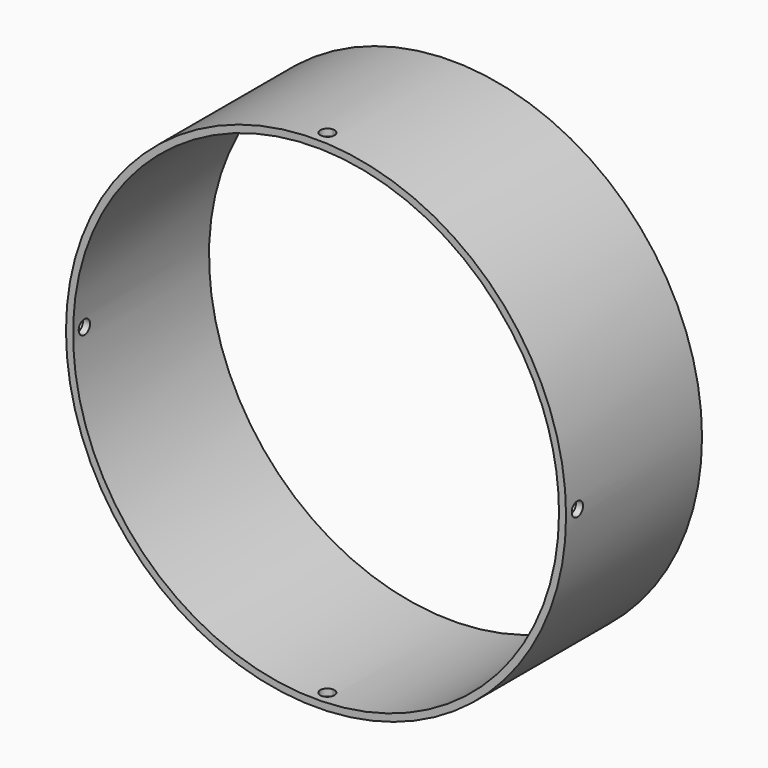
from build123d import *
from build123d import SkipClean  # not in build123d's __all__

# Parameters (mm, degrees)
F0_R     = 88.295
F1_DEPTH = 60
F2_R     = 2.5
F3_DEPTH = 300
F4_DEPTH = 300
F6_DEPTH = 300
F7_DEPTH = 300


with BuildPart() as f1:
    # F0 (on Front) → F1 (new body)
    with BuildSketch(Plane.XZ):
        Circle(F0_R)
        with BuildLine():
            ThreePointArc((80, 30.9964840748), (84.3338070557, 15.7667692474), (85.795, 0))
            ThreePointArc((85.795, 0), (-84.3338070557, -15.7667692474), (80, 30.9964840748))
        make_face(mode=Mode.SUBTRACT)
    extrude(amount=F1_DEPTH)

    # F2 (on Right) → F3 (cut)
    with BuildSketch(Plane.YZ):
        with Locations((-55, 0)):
            Circle(F2_R)
    extrude(amount=-F3_DEPTH, mode=Mode.SUBTRACT)

    # F2 (on Right) → F4 (cut)
    with BuildSketch(Plane.YZ):
        with Locations((-55, 0)):
            Circle(F2_R)
    with SkipClean():  # cleaning this boolean's faces spoils the solid; the shape is the same uncleaned
        extrude(amount=F4_DEPTH, mode=Mode.SUBTRACT)

    # F5 (on Top) → F6 (cut)
    with BuildSketch(Plane.XY):
        with BuildLine():
            ThreePointArc((0, -52.5), (-1.767766953, -56.767766953), (2.5, -55))
            ThreePointArc((2.5, -55), (1.767766953, -53.232233047), (0, -52.5))
        make_face()
    with SkipClean():  # cleaning this boolean's faces spoils the solid; the shape is the same uncleaned
        extrude(amount=-F6_DEPTH, mode=Mode.SUBTRACT)

    # F5 (on Top) → F7 (cut)
    with BuildSketch(Plane.XY):
        with BuildLine():
            ThreePointArc((0, -52.5), (-1.767766953, -56.767766953), (2.5, -55))
            ThreePointArc((2.5, -55), (1.767766953, -53.232233047), (0, -52.5))
        make_face()
    with SkipClean():  # cleaning this boolean's faces spoils the solid; the shape is the same uncleaned
        extrude(amount=F7_DEPTH, mode=Mode.SUBTRACT)


solid = f1.part
